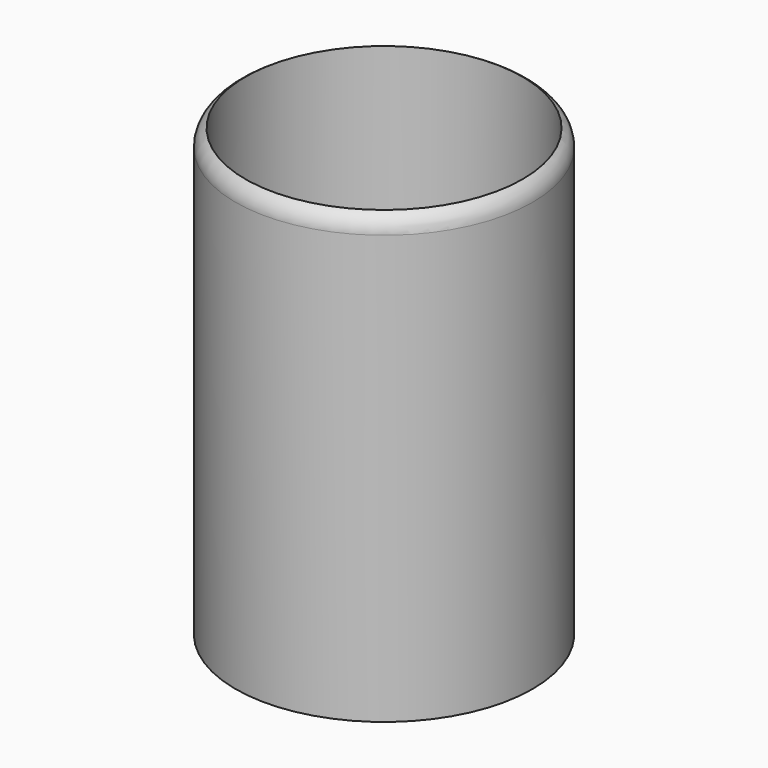
from build123d import *

# Parameters (mm, degrees)
F0_R     = 38.1
F1_DEPTH = 114.3
F2_T     = -2.54


# Not quite as in the source:
# - a fillet or chamfer that OpenCascade refuses, or shapes differently, is made with other operations: its cross-section is extruded or revolved along the edge and cut away or added


with BuildPart() as f1:
    # F0 (on Top) → F1 (new body)
    with BuildSketch(Plane.XY):
        Circle(F0_R)
    extrude(amount=F1_DEPTH)

    # F2
    f2_openings = [f1.faces().sort_by_distance(p)[0] for p in [
        (0, 0, 114.3),
    ]]
    offset(amount=F2_T, openings=f2_openings)

    # F3: fillet of radius 5.08 on 1 edges, made by hand

    # F3_s1 → F3_t2 (revolve, cut)
    with BuildSketch(Plane.XZ):
        with BuildLine():
            ThreePointArc((38.1, 109.9005909488), (37.4194090512, 112.4405909488), (35.56, 114.3))
            Line((35.56, 114.3), (38.1, 114.3))
            Line((38.1, 114.3), (38.1, 109.9005909488))
        make_face()
    revolve(axis=Axis((0, 0, 114.3), (0, 0, 1)), mode=Mode.SUBTRACT)


solid = f1.part
